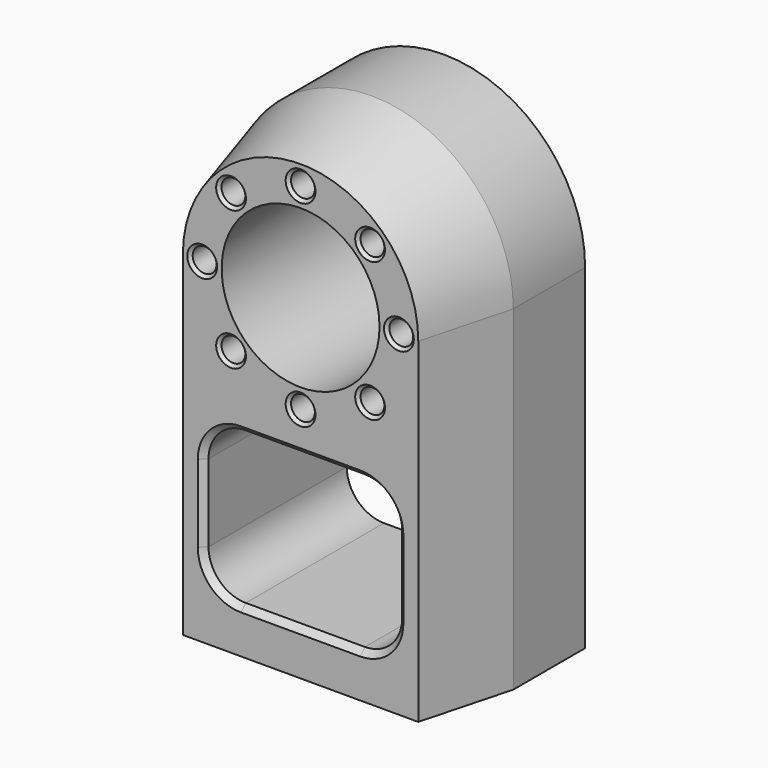
from build123d import *

# Parameters (mm, degrees)
F0_R     = 4
F0_R_2   = 26.5
F1_DEPTH = 60
F2_SIZE  = 1
F3_SIZE  = 2
F4_SIZE2 = 29.8564064606
F4_SIZE  = 8
F6_D     = 8.5
F6_DEPTH = 25
F6_TIP   = 2.5536576309


with BuildPart() as f1:
    # F0 (on Front) → F1 (new body)
    with BuildSketch(Plane.XZ):
        with BuildLine():
            Line((-45.9991587698, 54.2627746064), (-45.9991587698, -58.2372253936))
            Line((-45.9991587698, -58.2372253936), (49.0008412302, -58.2372253936))
            Line((49.0008412302, -58.2372253936), (49.0008412302, 54.2627746064))
            ThreePointArc((49.0008412302, 54.2627746064), (1.5008412302, 101.7627746064), (-45.9991587698, 54.2627746064))
        make_face()
        with BuildLine():
            ThreePointArc((-30.9991587698, -4.7372253936), (-27.3379935347, 4.1016093712), (-18.4991587698, 7.7627746064))
            Line((-18.4991587698, 7.7627746064), (21.5008412302, 7.7627746064))
            ThreePointArc((21.5008412302, 7.7627746064), (30.339675995, 4.1016093712), (34.0008412302, -4.7372253936))
            Line((34.0008412302, -4.7372253936), (34.0008412302, -30.7372253936))
            ThreePointArc((34.0008412302, -30.7372253936), (30.339675995, -39.5760601585), (21.5008412302, -43.2372253936))
            Line((21.5008412302, -43.2372253936), (-18.4991587698, -43.2372253936))
            ThreePointArc((-18.4991587698, -43.2372253936), (-27.3379935347, -39.5760601585), (-30.9991587698, -30.7372253936))
            Line((-30.9991587698, -30.7372253936), (-30.9991587698, -4.7372253936))
        make_face(mode=Mode.SUBTRACT)
        with Locations((1.5008412302, 21.2627746064)):
            Circle(F0_R, mode=Mode.SUBTRACT)
        with Locations((-31.4991587698, 54.2627746064)):
            Circle(F0_R, mode=Mode.SUBTRACT)
        with Locations((-21.833682549, 30.9282508272)):
            Circle(F0_R, mode=Mode.SUBTRACT)
        with Locations((1.5008412302, 54.2627746064)):
            Circle(F0_R_2, mode=Mode.SUBTRACT)
        with Locations((-21.833682549, 77.5972983855)):
            Circle(F0_R, mode=Mode.SUBTRACT)
        with Locations((1.5008412302, 87.2627746064)):
            Circle(F0_R, mode=Mode.SUBTRACT)
        with Locations((24.8353650093, 30.9282508272)):
            Circle(F0_R, mode=Mode.SUBTRACT)
        with Locations((34.5008412302, 54.2627746064)):
            Circle(F0_R, mode=Mode.SUBTRACT)
        with Locations((24.8353650093, 77.5972983855)):
            Circle(F0_R, mode=Mode.SUBTRACT)
    extrude(amount=F1_DEPTH)

    # F2
    f2_edges = [f1.edges().sort_by_distance(p)[0] for p in [
        (-35.499159, -60, 54.262775),
        (-25.833683, -60, 77.597298),
        (-2.499159, -60, 87.262775),
        (20.835365, -60, 77.597298),
        (30.500841, -60, 54.262775),
        (20.835365, -60, 30.928251),
        (-2.499159, -60, 21.262775),
        (-25.833683, -60, 30.928251),
    ]]
    chamfer(f2_edges, length=F2_SIZE)

    # F3
    f3_edges = [f1.edges().sort_by_distance(p)[0] for p in [
        (1.500841, -60, 7.762775),
    ]]
    chamfer(f3_edges, length=F3_SIZE)

    # F4
    f4_edges = [f1.edges().sort_by_distance(p)[0] for p in [
        (1.500841, -60, 101.762775),
    ]]
    f4_side = f1.faces().sort_by_distance((1.500841, -60, 11.623554))[0]
    chamfer(f4_edges, length=F4_SIZE, length2=F4_SIZE2, reference=f4_side)

    # F6
    with Locations(Plane(origin=(0, 0, -58.2372253936), x_dir=(1, 0, 0), z_dir=(0, 0, -1))):
        with Locations((-35.9991587698, 25), (39.0008412302, 25)):
            Hole(F6_D / 2, depth=F6_DEPTH)
            with Locations((0, 0, -(F6_DEPTH + F6_TIP / 2))):  # 118° drill point
                Cone(0, F6_D / 2, F6_TIP, mode=Mode.SUBTRACT)


solid = f1.part
